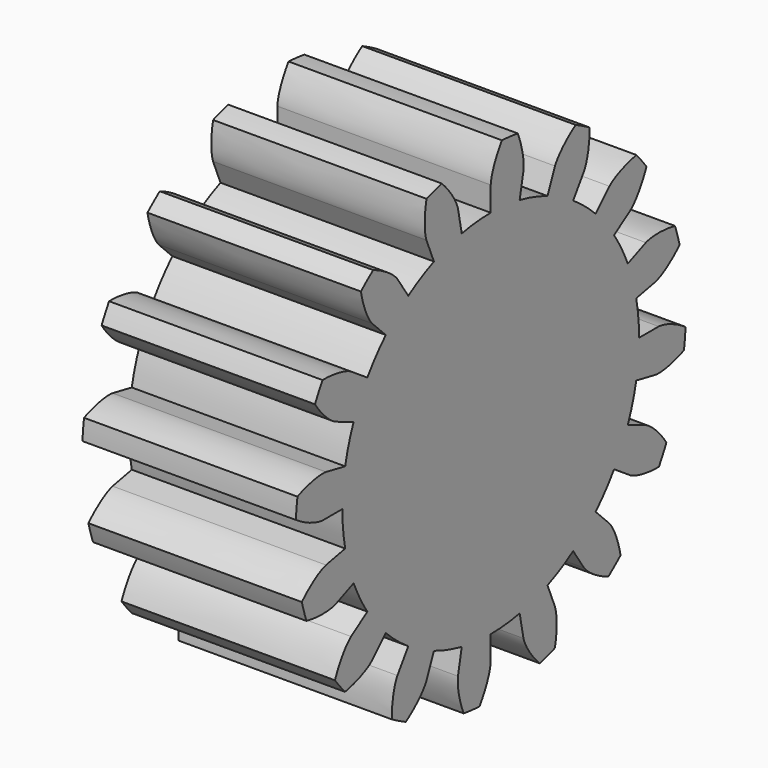
from build123d import *

# Parameters (mm, degrees)
F3_DEPTH        = 10
F3_COPIES_COUNT = 16


# Not quite as in the source:
# - a feature of the source that left no trace in its solid (it failed there, or was rolled back) is left out
# - a pattern or mirror of a feature is missing from the dataset's text; its kind, count and spacing are read off the source's solid
# - a feature names something its author has since deleted; it is built from what else it names


with BuildPart() as f3:
    # F2 (on Right) → F3 (new body)
    with BuildSketch(Plane.YZ):
        with BuildLine():
            ThreePointArc((-8.69061, 0), (0, -8.69061), (8.69061, 0))
            ThreePointArc((8.69061, 0), (0.8518287399, 8.6487623375), (-8.5236223657, 1.6954539034))
            ThreePointArc((-8.5236223657, 1.6954539034), (-8.6487623375, 0.8518287399), (-8.69061, 0))
        make_face()
        with BuildLine():
            ThreePointArc((-8.69061, 0), (-8.6487623375, 0.8518287399), (-8.5236223657, 1.6954539034))
            Line((-8.5236223657, 1.6954539034), (-9.6473767422, 1.9189825468))
            add(Edge.make_bspline(
                [(-9.6473767422, 1.9189825468), (-9.6530150918, 1.9201040843), (-9.658835549, 1.9209090829), (-9.6997192414, 1.9262346756), (-9.7590493996, 1.9302321478), (-9.8457579314, 1.9321979375), (-9.9561730838, 1.9289838059), (-10.0911080115, 1.9183659751), (-10.2496438085, 1.89785302), (-10.4312331312, 1.8650519276), (-10.6347392824, 1.8177340758), (-10.8599631052, 1.7531526547), (-11.0876841257, 1.6759336994), (-11.2484008704, 1.6120335571), (-11.3199340913, 1.5824007611)],
                knots=[0, 0, 0, 0, 0.0202164122, 0.055231725, 0.1004362437, 0.1539229332, 0.2145711301, 0.2816202297, 0.3545102827, 0.4328067574, 0.5161597183, 0.6042794907, 0.6969211254, 0.7772279414, 0.7772279414, 0.7772279414, 0.7772279414], degree=3))
            ThreePointArc((-11.3199340913, 1.5824007611), (-11.3749614259, 1.120335914), (-11.4111358059, 0.6564142129))
            add(Edge.make_bspline(
                [(-9.8363800262, 0), (-9.8421288376, 0), (-9.8479945038, 0.0003459841), (-9.8891315991, 0.0030987338), (-9.9481016132, 0.0107528116), (-10.0335275713, 0.0257407894), (-10.1411940816, 0.05043409), (-10.2714648364, 0.0871724007), (-10.4229525336, 0.1382200047), (-10.5946534927, 0.2058171528), (-10.7850180753, 0.2919278859), (-10.9933150753, 0.3992073813), (-11.2015958293, 0.5193687632), (-11.3467581475, 0.6133953637), (-11.4111358059, 0.6564142129)],
                knots=[0, 0, 0, 0, 0.0202164122, 0.055231725, 0.1004362437, 0.1539229332, 0.2145711301, 0.2816202297, 0.3545102827, 0.4328067574, 0.5161597183, 0.6042794907, 0.6969211254, 0.7772279414, 0.7772279414, 0.7772279414, 0.7772279414], degree=3))
            Line((-9.8363800262, 0), (-8.69061, 0))
        make_face()
    extrude(amount=F3_DEPTH)

    # F3_copies: F3 ×16 about axis
    f3_copies_axis = Axis((0, 0, 0), (1, 0, 0))


with BuildPart() as f3_1:
    add(f3.part)
    for i in range(1, F3_COPIES_COUNT):
        add(f3.part.rotate(f3_copies_axis, i * 360 / F3_COPIES_COUNT))


solid = f3_1.part
